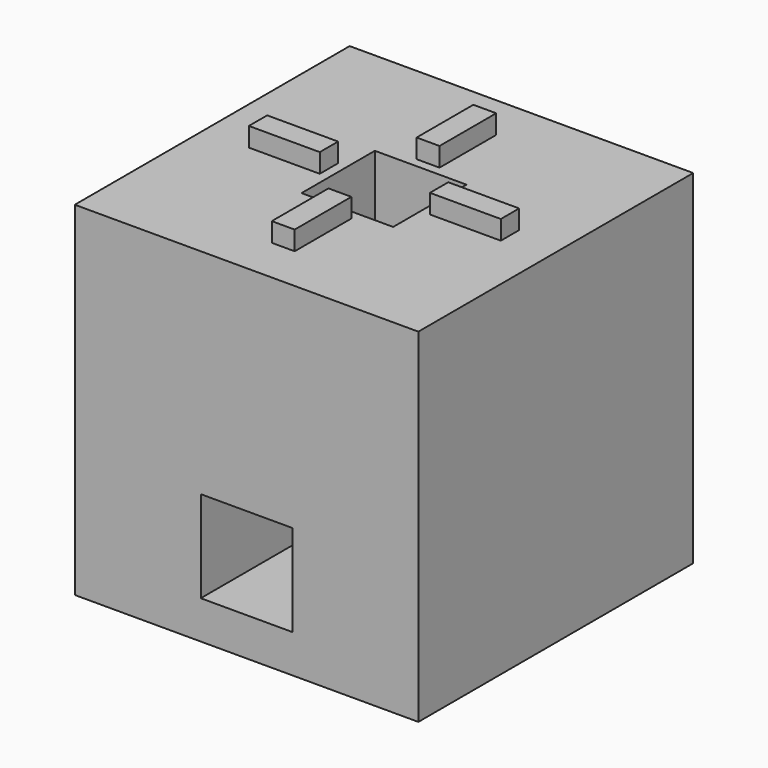
from build123d import *

# Parameters (mm, degrees)
F0_W          = 914.4
F0_H          = 914.4
F1_DEPTH      = 914.4
F2_W          = 243.84
F2_H          = 243.84
F3_DEPTH      = 335.28
F4_W          = 243.84
F4_H          = 243.84
F5_DEPTH      = 812.9016
F6_W          = 188.6856555939
F6_H          = 60.96
F6_W_2        = 60.96
F6_H_2        = 188.6712
F7_DEPTH      = 50.81016
F7_DEPTH_BACK = 30.48


# Not quite as in the source:
# - a feature names something its author has since deleted; it is built from what else it names


with BuildPart() as f1:
    # F0 (on Front) → F1 (new body)
    with BuildSketch(Plane.XZ):
        Rectangle(F0_W, F0_H)
    extrude(amount=F1_DEPTH)

    # F2 (on face) → F3 (cut)
    with BuildSketch(Plane.XZ.offset(914.4)):
        with Locations((0, -233.7816)):
            Rectangle(F2_W, F2_H)
    extrude(amount=-F3_DEPTH, mode=Mode.SUBTRACT)

    # F4 (on face) → F5 (cut)
    with BuildSketch(Plane.XY.offset(457.2)):
        with Locations((0, -457.2)):
            Rectangle(F4_W, F4_H)
    extrude(amount=-F5_DEPTH, mode=Mode.SUBTRACT)

    # F6 (on face) → F7 (join, two sides)
    with BuildSketch(Plane.XY.offset(457.2)) as f7_sk:
        with Locations((240.9371722031, -457.2)):
            Rectangle(F6_W, F6_H)
        with Locations((0, -216.2556)):
            Rectangle(F6_W_2, F6_H_2)
        with Locations((-240.9371722031, -457.2)):
            Rectangle(F6_W, F6_H)
        with Locations((0, -698.1444)):
            Rectangle(F6_W_2, F6_H_2)
    extrude(amount=F7_DEPTH)
    extrude(f7_sk.sketch, amount=-F7_DEPTH_BACK)


solid = f1.part
